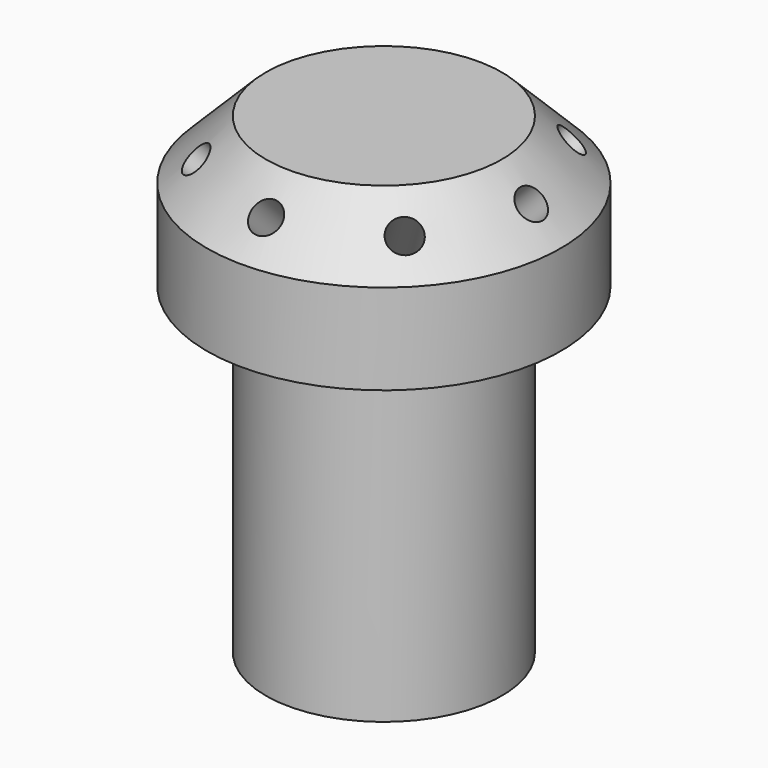
from build123d import *

# Parameters (mm, degrees)
F5_COPIES_COUNT = 8


# Not quite as in the source:
# - a pattern or mirror of a feature is missing from the dataset's text; its kind, count and spacing are read off the source's solid


with BuildPart() as f1:
    # F0 (on Front) → F1 (revolve)
    with BuildSketch(Plane.XZ):
        Polygon((0, -76.2), (0, 0), (-19.05, 0), (-28.575, -9.525), (-28.575, -24.13), (-19.05, -24.13), (-19.05, -76.2), align=None)
    revolve(axis=Axis((0, 0, -1.7110773744), (0, 0, -1)))

    # F2 (on Front) → F3 (revolve, cut)
    with BuildSketch(Plane.XZ):
        with BuildLine():
            ThreePointArc((0, -14.605), (-8.9802561211, -18.3247438789), (-12.7, -27.305))
            Line((-12.7, -27.305), (-12.7, -76.2))
            Line((-12.7, -76.2), (0, -76.2))
            Line((0, -76.2), (0, -14.605))
        make_face()
    revolve(axis=Axis((0, 0, -45.4025), (0, 0, -1)), mode=Mode.SUBTRACT)

    # F4 (on Front) → F5 (revolve, cut)
    with BuildSketch(Plane.XZ):
        Polygon((-23.8125, -4.7625), (-25.6085512242, -6.5585512242), (-7.6480389821, -24.5190634664), (-5.8519877579, -22.7230122421), align=None)
    f5 = revolve(axis=Axis((-14.8322438789, 0, -13.7427561211), (0.7071067812, 0, -0.7071067812)), mode=Mode.SUBTRACT)

    # F5_copies: F5 ×8 about axis
    f5_copies_axis = Axis((0, 0, 0), (0, 0, 1))
    for i in range(1, F5_COPIES_COUNT):
        add(f5.rotate(f5_copies_axis, i * 360 / F5_COPIES_COUNT), mode=Mode.SUBTRACT)


solid = f1.part
